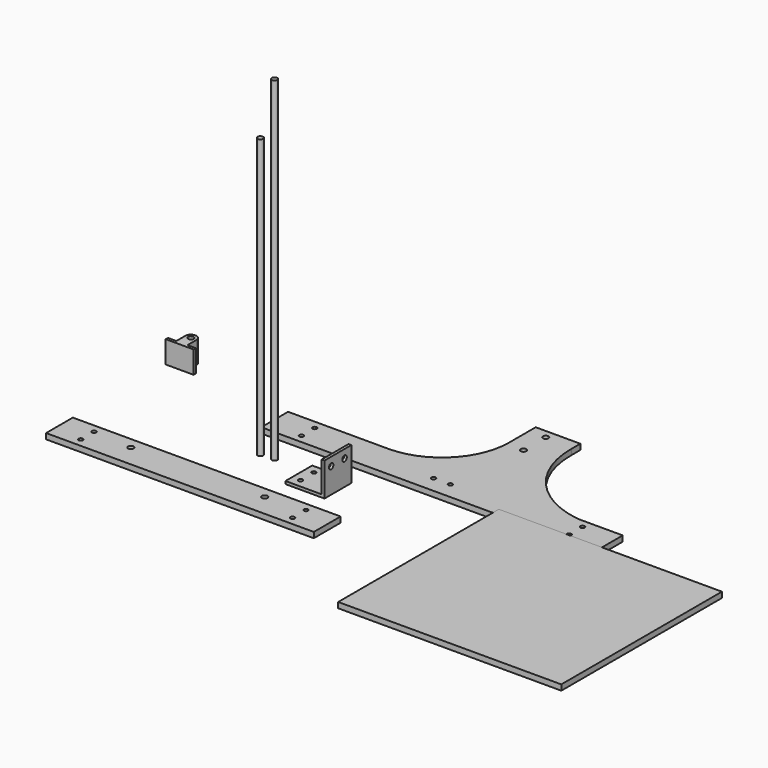
from build123d import *

# Parameters (mm, degrees)
F0_W      = 609.6
F0_H      = 76.2
F1_DEPTH  = 12.7
F3_DEPTH  = 12.7
F5_D      = 9.652
F5_DEPTH  = 25.4
F5_TIP    = 2.8997533474
F7_D      = 9.652
F7_DEPTH  = 25.4
F7_TIP    = 2.8997533474
F8_D      = 9.652
F8_DEPTH  = 25.4
F8_TIP    = 2.8997533474
F10_D     = 9.652
F10_DEPTH = 25.4
F10_TIP   = 2.8997533474
F12_D     = 12.7
F12_DEPTH = 25.4
F12_TIP   = 3.8154649308
F13_R     = 6.35
F14_DEPTH = 635
F15_D     = 12.7
F15_DEPTH = 25.4
F15_TIP   = 3.8154649308
F16_R     = 6.35
F17_DEPTH = 762
F18_W     = 69.85
F18_H     = 76.2
F18_W_2   = 6.35
F19_DEPTH = 6.35
F20_DEPTH = 69.85
F22_D     = 12.7
F22_DEPTH = 25.4
F22_TIP   = 3.8154649308
F23_D     = 12.7
F23_DEPTH = 25.4
F23_TIP   = 3.8154649308
F24_W     = 508
F24_H     = 457.2
F25_DEPTH = 12.7
F26_R     = 6.35
F27_DEPTH = 50.8
F28_DEPTH = 12.7
F30_D     = 9.652
F30_DEPTH = 25.4
F30_TIP   = 2.8997533474


# Not quite as in the source:
# - a feature names something its author has since deleted; it is built from what else it names


with BuildPart() as f1:
    # F0 (on Top) → F1 (new body)
    with BuildSketch(Plane.XY):
        with Locations((-91.9581856579, -223.2227385089)):
            Rectangle(F0_W, F0_H)
    extrude(amount=F1_DEPTH)

    # F5
    with Locations(Plane.XY.offset(12.7)):
        with Locations((149.3418143421, -242.2727385089), (149.3418143421, -204.1727385089)):
            Hole(F5_D / 2, depth=F5_DEPTH)
            with Locations((0, 0, -(F5_DEPTH + F5_TIP / 2))):  # 118° drill point
                Cone(0, F5_D / 2, F5_TIP, mode=Mode.SUBTRACT)

    # F8
    with Locations(Plane.XY.offset(12.7)):
        with Locations((-333.2581856579, -204.1727385089), (-333.2581856579, -242.2727385089)):
            Hole(F8_D / 2, depth=F8_DEPTH)
            with Locations((0, 0, -(F8_DEPTH + F8_TIP / 2))):  # 118° drill point
                Cone(0, F8_D / 2, F8_TIP, mode=Mode.SUBTRACT)

    # F15
    with Locations(Plane.XY.offset(12.7)):
        with Locations((-244.3581856579, -210.5227385089), (60.4418143421, -210.5227385089)):
            Hole(F15_D / 2, depth=F15_DEPTH)
            with Locations((0, 0, -(F15_DEPTH + F15_TIP / 2))):  # 118° drill point
                Cone(0, F15_D / 2, F15_TIP, mode=Mode.SUBTRACT)


with BuildPart() as f3:
    # F2 (on Top) → F3 (new body)
    with BuildSketch(Plane.XY):
        with BuildLine():
            Line((116.7021817187, 71.3612283528), (-111.8978182813, 71.3612283528))
            Line((-111.8978182813, 71.3612283528), (-111.8978182813, -4.8387716472))
            Line((-111.8978182813, -4.8387716472), (650.1021817187, -4.8387716472))
            Line((650.1021817187, -4.8387716472), (650.1021817187, 71.3612283528))
            Line((650.1021817187, 71.3612283528), (548.5021817187, 71.3612283528))
            ThreePointArc((548.5021817187, 71.3612283528), (420.9723533293, 139.160128512), (370.7021817187, 274.5612283528))
            Line((370.7021817187, 274.5612283528), (370.7021817187, 299.9612283528))
            Line((370.7021817187, 299.9612283528), (269.1021817187, 299.9612283528))
            Line((269.1021817187, 299.9612283528), (269.1021817187, 223.7612283528))
            ThreePointArc((269.1021817187, 223.7612283528), (224.4652551716, 115.9981549), (116.7021817187, 71.3612283528))
        make_face()
    extrude(amount=F3_DEPTH)

    # F7
    with Locations(Plane.XY.offset(12.7)):
        with Locations((-35.6978182813, 52.3112283528), (-35.6978182813, 14.2112283528), (573.9021817187, 52.3112283528), (573.9021817187, 14.2112283528)):
            Hole(F7_D / 2, depth=F7_DEPTH)
            with Locations((0, 0, -(F7_DEPTH + F7_TIP / 2))):  # 118° drill point
                Cone(0, F7_D / 2, F7_TIP, mode=Mode.SUBTRACT)

    # F10
    with Locations(Plane.XY.offset(12.7)):
        with Locations((288.1521817187, 33.2612283528), (250.0521817187, 33.2612283528)):
            Hole(F10_D / 2, depth=F10_DEPTH)
            with Locations((0, 0, -(F10_DEPTH + F10_TIP / 2))):  # 118° drill point
                Cone(0, F10_D / 2, F10_TIP, mode=Mode.SUBTRACT)

    # F12
    with Locations(Plane.XY.offset(12.7)):
        with Locations((307.2021817187, 217.4112283528)):
            Hole(F12_D / 2, depth=F12_DEPTH)
            with Locations((0, 0, -(F12_DEPTH + F12_TIP / 2))):  # 118° drill point
                Cone(0, F12_D / 2, F12_TIP, mode=Mode.SUBTRACT)

    # F23
    with Locations(Plane.XY.offset(12.7)):
        with Locations((307.2021817187, 280.9112283528)):
            Hole(F23_D / 2, depth=F23_DEPTH)
            with Locations((0, 0, -(F23_DEPTH + F23_TIP / 2))):  # 118° drill point
                Cone(0, F23_D / 2, F23_TIP, mode=Mode.SUBTRACT)


with BuildPart() as f14:
    # F13 (on Top) → F14 (new body)
    with BuildSketch(Plane.XY):
        with Locations((-62.5835806131, -69.0215006471)):
            Circle(F13_R)
    extrude(amount=F14_DEPTH)


with BuildPart() as f17:
    # F16 (on Top) → F17 (new body)
    with BuildSketch(Plane.XY):
        with Locations((-32.141212374, -66.7899250984)):
            Circle(F16_R)
    extrude(amount=F17_DEPTH)


with BuildPart() as f19:
    # F18 (on Top) → F19 (new body)
    with BuildSketch(Plane.XY):
        with Locations((83.3102070808, -82.4468559648)):
            Rectangle(F18_W, F18_H)
        with Locations((121.4102070808, -82.4468559648)):
            Rectangle(F18_W_2, F18_H)
    extrude(amount=-F19_DEPTH)

    # F18 (on Top) → F20 (join)
    with BuildSketch(Plane.XY):
        with Locations((121.4102070808, -82.4468559648)):
            Rectangle(F18_W_2, F18_H)
    extrude(amount=F20_DEPTH)

    # F22
    with Locations(Plane.YZ.offset(124.5852070808)):
        with Locations((-101.4968559648, 50.8), (-63.3968559648, 50.8)):
            Hole(F22_D / 2, depth=F22_DEPTH)
            with Locations((0, 0, -(F22_DEPTH + F22_TIP / 2))):  # 118° drill point
                Cone(0, F22_D / 2, F22_TIP, mode=Mode.SUBTRACT)

    # F28 (add): a face of the model
    f28_faces = [f19.faces().sort_by_distance(p)[0] for p in [
        (48.3852070808, -82.4468559648, -3.175),
    ]]
    extrude(f28_faces, amount=F28_DEPTH)

    # F30
    with Locations(Plane.XY):
        with Locations((54.7352070808, -63.3968559648), (54.7352070808, -101.4968559648)):
            Hole(F30_D / 2, depth=F30_DEPTH)
            with Locations((0, 0, -(F30_DEPTH + F30_TIP / 2))):  # 118° drill point
                Cone(0, F30_D / 2, F30_TIP, mode=Mode.SUBTRACT)


with BuildPart() as f25:
    # F24 (on Top) → F25 (new body)
    with BuildSketch(Plane.XY):
        with Locations((669.1857836282, -216.2299761653)):
            Rectangle(F24_W, F24_H)
    extrude(amount=F25_DEPTH)


with BuildPart() as f27:
    # F26 (on Top) → F27 (new body)
    with BuildSketch(Plane.XY):
        with BuildLine():
            Line((-410.6456120811, 102.9733254265), (-410.6456120811, 96.6233254265))
            Line((-410.6456120811, 96.6233254265), (-347.1456120811, 96.6233254265))
            Line((-347.1456120811, 96.6233254265), (-347.1456120811, 102.9733254265))
            Line((-347.1456120811, 102.9733254265), (-366.1956120811, 102.9733254265))
            Line((-366.1956120811, 102.9733254265), (-366.1956120811, 128.3733254265))
            ThreePointArc((-366.1956120811, 128.3733254265), (-369.9153559601, 137.3535815476), (-378.8956120811, 141.0733254265))
            ThreePointArc((-378.8956120811, 141.0733254265), (-387.8758682022, 137.3535815476), (-391.5956120811, 128.3733254265))
            Line((-391.5956120811, 128.3733254265), (-391.5956120811, 102.9733254265))
            Line((-391.5956120811, 102.9733254265), (-410.6456120811, 102.9733254265))
        make_face()
        with Locations((-378.8956120811, 128.3733254265)):
            Circle(F26_R, mode=Mode.SUBTRACT)
    extrude(amount=F27_DEPTH)


solid = Compound([f1.part, f3.part, f14.part, f17.part, f19.part, f25.part, f27.part])
